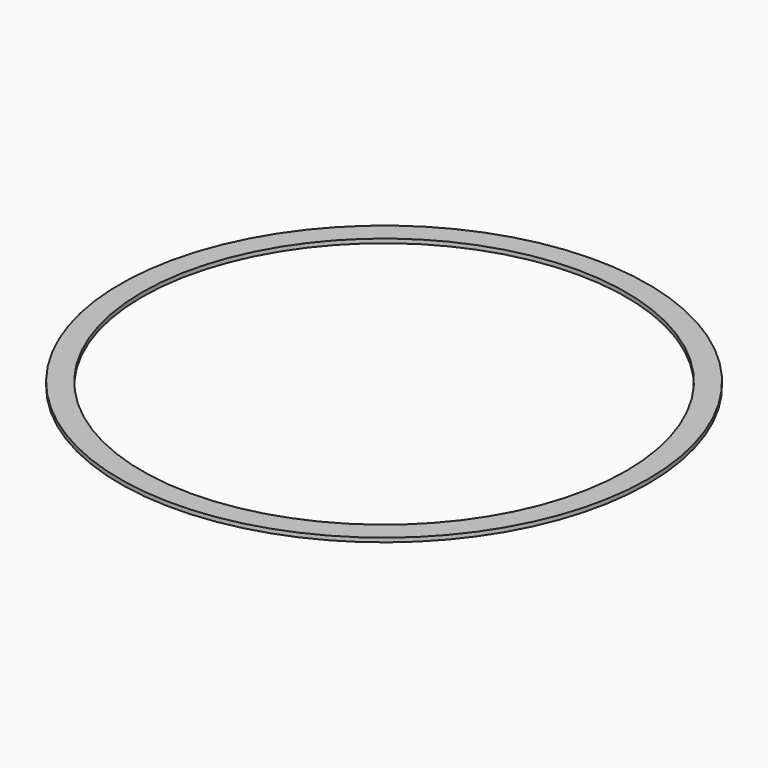
from build123d import *

# Parameters (mm, degrees)
F0_R     = 305.14417
F0_R_2   = 279.74417
F1_DEPTH = 4.7625


# Not quite as in the source:
# - a length typed as a fraction of an inch, garbled in the dataset ("3 / 203.2 mm" for 3/8 in), is restored


with BuildPart() as f1:
    # F0 (on Top) → F1 (new body)
    with BuildSketch(Plane.XY):
        Circle(F0_R)
        Circle(F0_R_2, mode=Mode.SUBTRACT)
    extrude(amount=F1_DEPTH)


solid = f1.part
